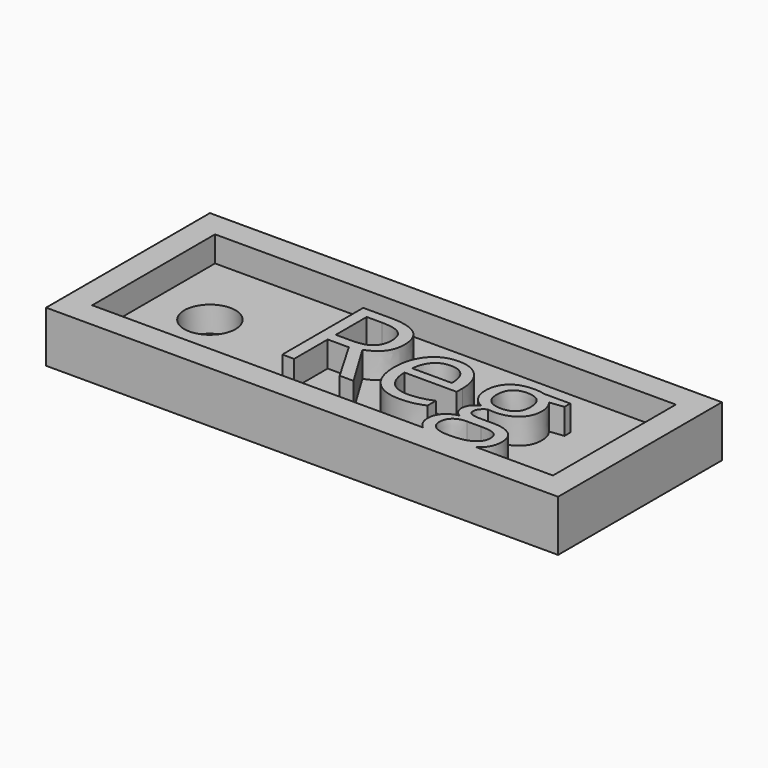
from build123d import *

# Parameters (mm, degrees)
F0_W         = 63.5
F0_H         = 25.4
F1_DEPTH     = 6.35
F2_W         = 57.15
F2_H         = 19.05
F3_DEPTH     = 3.175
F4_TEXT_SIZE = 17.5643259556
F5_DEPTH     = 3.175
F6_R         = 3.175
F7_DEPTH     = 3.176


# Not quite as in the source:
# - Text() gives the source's letters only with a copy of the font that has no kerning and outlines rounded to 1/6400 em; it was checked with that copy


with BuildPart() as f1:
    # F0 (on Top) → F1 (new body)
    with BuildSketch(Plane.XY):
        Rectangle(F0_W, F0_H)
    extrude(amount=F1_DEPTH)

    # F2 (on face) → F3 (cut)
    with BuildSketch(Plane.XY.offset(6.35)):
        Rectangle(F2_W, F2_H)
    extrude(amount=-F3_DEPTH, mode=Mode.SUBTRACT)

    # F4 (on face) → F5 (join)
    with BuildSketch(Plane.XY.offset(3.175)):
        with Locations((-9.4631686807, -6.0882298276)):
            Text('Reg', F4_TEXT_SIZE, font='Open Sans', text_align=(TextAlign.LEFT, TextAlign.BOTTOM))
    extrude(amount=F5_DEPTH)

    # F6 (on face) → F7 (cut, through all)
    with BuildSketch(Plane.XY.offset(3.175)):
        with Locations((-21.59, 0)):
            Circle(F6_R)
    extrude(amount=-F7_DEPTH, mode=Mode.SUBTRACT)


solid = f1.part
